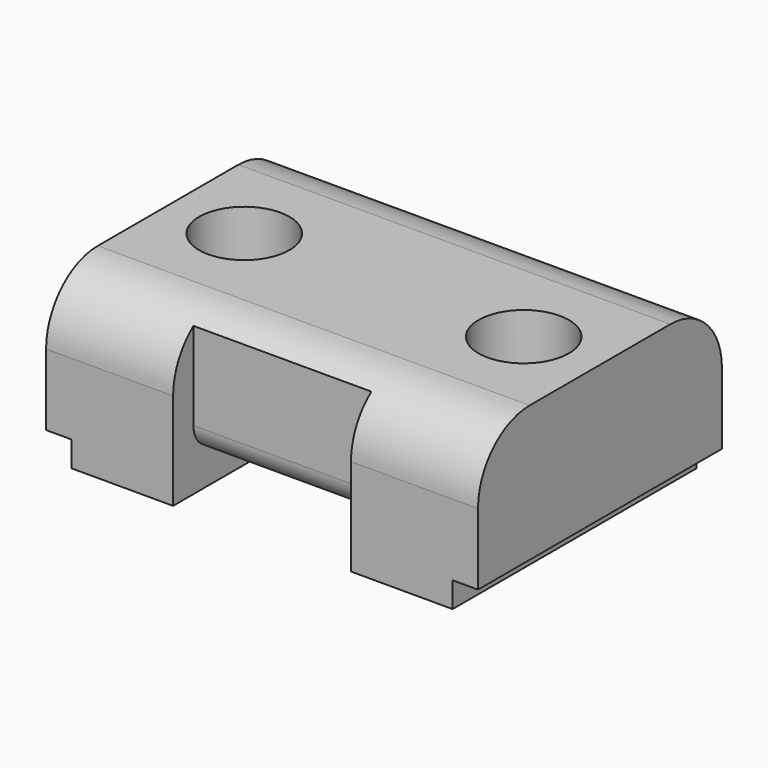
from build123d import *

# Parameters (mm, degrees)
F0_W      = 12
F0_H      = 6.35
F1_DEPTH  = 4
F3_DEPTH  = 7
F4_W      = 12
F4_H      = 6.35
F5_DEPTH  = 4
F6_R      = 1.778
F7_DEPTH  = 25.4
F8_W      = 12
F8_H      = 5.35
F9_DEPTH  = 1
F10_W     = 12
F10_H     = 5.35
F11_DEPTH = 1
F12_F1_R  = 2.54
F12_F2_R  = 2.54


with BuildPart() as f1:
    # F0 (on Right) → F1 (new body)
    with BuildSketch(Plane.YZ):
        with Locations((6, 3.175)):
            Rectangle(F0_W, F0_H)
    extrude(amount=F1_DEPTH)

    # F2 (on face) → F3 (join)
    with BuildSketch(Plane.YZ.offset(4)):
        with BuildLine():
            ThreePointArc((10.2598245749, 1.38), (10.3587316459, 1.3427714117), (10.4085431086, 1.2495652174))
            ThreePointArc((10.4085431086, 1.2495652174), (10.4423882857, 1.091937846), (10.5011235955, 0.9417977528))
            ThreePointArc((10.5011235955, 0.9417977528), (11, 0.63), (11.4988764045, 0.9417977528))
            ThreePointArc((11.4988764045, 0.9417977528), (11.5576117143, 1.091937846), (11.5914568914, 1.2495652174))
            ThreePointArc((11.5914568914, 1.2495652174), (11.6412683541, 1.3427714117), (11.7401754251, 1.38))
            Line((11.7401754251, 1.38), (12, 1.38))
            Line((12, 1.38), (12, 6.35))
            Line((12, 6.35), (1, 6.35))
            Line((1, 6.35), (1, 2.38))
            ThreePointArc((1, 2.38), (1.2928932188, 1.6728932188), (2, 1.38))
            Line((2, 1.38), (2.2598245749, 1.38))
            ThreePointArc((2.2598245749, 1.38), (2.3587316459, 1.3427714117), (2.4085431086, 1.2495652174))
            ThreePointArc((2.4085431086, 1.2495652174), (2.4423882857, 1.091937846), (2.5011235955, 0.9417977528))
            ThreePointArc((2.5011235955, 0.9417977528), (3, 0.63), (3.4988764045, 0.9417977528))
            ThreePointArc((3.4988764045, 0.9417977528), (3.5576117143, 1.091937846), (3.5914568914, 1.2495652174))
            ThreePointArc((3.5914568914, 1.2495652174), (3.6412683541, 1.3427714117), (3.7401754251, 1.38))
            Line((3.7401754251, 1.38), (4, 1.38))
            Line((4, 1.38), (4.2598245749, 1.38))
            ThreePointArc((4.2598245749, 1.38), (4.3587316459, 1.3427714117), (4.4085431086, 1.2495652174))
            ThreePointArc((4.4085431086, 1.2495652174), (4.4423882857, 1.091937846), (4.5011235955, 0.9417977528))
            ThreePointArc((4.5011235955, 0.9417977528), (5, 0.63), (5.4988764045, 0.9417977528))
            ThreePointArc((5.4988764045, 0.9417977528), (5.5576117143, 1.091937846), (5.5914568914, 1.2495652174))
            ThreePointArc((5.5914568914, 1.2495652174), (5.6412683541, 1.3427714117), (5.7401754251, 1.38))
            Line((5.7401754251, 1.38), (6, 1.38))
            Line((6, 1.38), (6.2598245749, 1.38))
            ThreePointArc((6.2598245749, 1.38), (6.3587316459, 1.3427714117), (6.4085431086, 1.2495652174))
            ThreePointArc((6.4085431086, 1.2495652174), (6.4423882857, 1.091937846), (6.5011235955, 0.9417977528))
            ThreePointArc((6.5011235955, 0.9417977528), (7, 0.63), (7.4988764045, 0.9417977528))
            ThreePointArc((7.4988764045, 0.9417977528), (7.5576117143, 1.091937846), (7.5914568914, 1.2495652174))
            ThreePointArc((7.5914568914, 1.2495652174), (7.6412683541, 1.3427714117), (7.7401754251, 1.38))
            Line((7.7401754251, 1.38), (8, 1.38))
            Line((8, 1.38), (8.2598245749, 1.38))
            ThreePointArc((8.2598245749, 1.38), (8.3587316459, 1.3427714117), (8.4085431086, 1.2495652174))
            ThreePointArc((8.4085431086, 1.2495652174), (8.4423882857, 1.091937846), (8.5011235955, 0.9417977528))
            ThreePointArc((8.5011235955, 0.9417977528), (9, 0.63), (9.4988764045, 0.9417977528))
            ThreePointArc((9.4988764045, 0.9417977528), (9.5576117143, 1.091937846), (9.5914568914, 1.2495652174))
            ThreePointArc((9.5914568914, 1.2495652174), (9.6412683541, 1.3427714117), (9.7401754251, 1.38))
            Line((9.7401754251, 1.38), (10, 1.38))
            Line((10, 1.38), (10.2598245749, 1.38))
        make_face()
    extrude(amount=F3_DEPTH)

    # F4 (on face) → F5 (join)
    with BuildSketch(Plane.YZ.offset(11)):
        with Locations((6, 3.175)):
            Rectangle(F4_W, F4_H)
    extrude(amount=F5_DEPTH)

    # F6 (on face) → F7 (cut)
    with BuildSketch(Plane.XY.offset(6.35)):
        with Locations((2, 6)):
            Circle(F6_R)
        with Locations((13, 6)):
            Circle(F6_R)
    extrude(amount=-F7_DEPTH, mode=Mode.SUBTRACT)

    # F8 (on face) → F9 (join)
    with BuildSketch(Plane(origin=(0, 0, 0), x_dir=(0, -1, 0), z_dir=(-1, 0, 0))):
        with Locations((-6, 3.675)):
            Rectangle(F8_W, F8_H)
    extrude(amount=F9_DEPTH)

    # F10 (on face) → F11 (join)
    with BuildSketch(Plane.YZ.offset(15)):
        with Locations((6, 3.675)):
            Rectangle(F10_W, F10_H)
    extrude(amount=F11_DEPTH)

    # F12: fillet of radius 2.54 on 3 edges, made by hand

    # F12_f1
    f12_f1_edges = [f1.edges().sort_by_distance(p)[0] for p in [
        (1.5, 0, 6.35),
    ]]
    fillet(f12_f1_edges, radius=F12_F1_R)

    # F12_f2
    f12_f2_edges = [f1.edges().sort_by_distance(p)[0] for p in [
        (7.5, 12, 6.35),
    ]]
    fillet(f12_f2_edges, radius=F12_F2_R)


solid = f1.part
